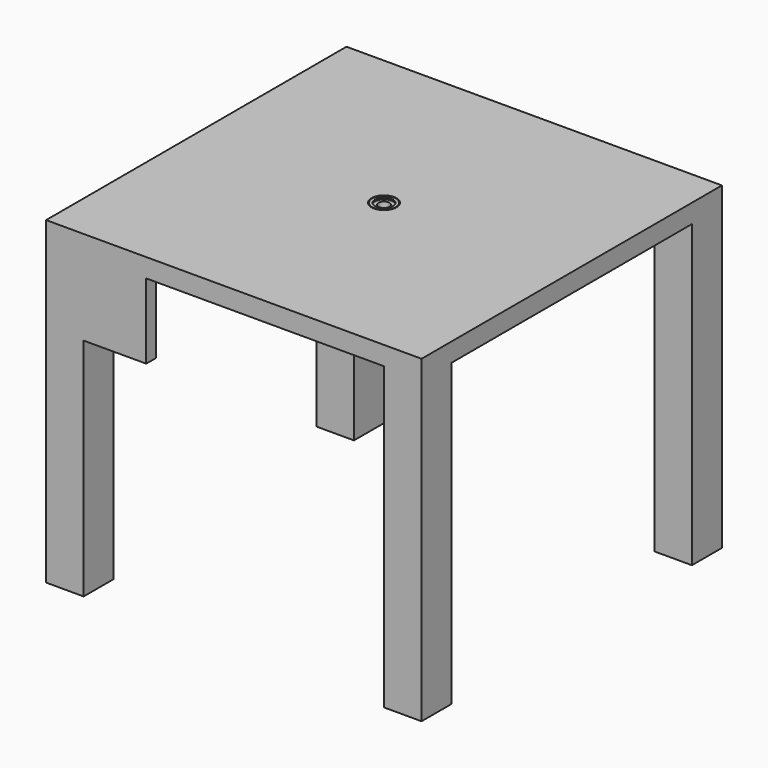
from build123d import *

# Parameters (mm, degrees)
F0_W      = 762
F0_H      = 762
F1_DEPTH  = 38.1
F2_W      = 76.2
F2_H      = 76.2
F3_DEPTH  = 609.6
F4_R      = 18.25625
F5_DEPTH  = 3.60934
F6_R      = 11.1125
F7_DEPTH  = 644.09166
F9_R      = 25.4
F9_R_2    = 23.8125
F10_DEPTH = 12.7
F11_W     = 127
F11_H     = 152.4
F12_DEPTH = 25.4


# Not quite as in the source:
# - a feature of the source that left no trace in its solid (it failed there, or was rolled back) is left out


with BuildPart() as f1:
    # F0 (on Top) → F1 (new body)
    with BuildSketch(Plane.XY):
        Rectangle(F0_W, F0_H)
    extrude(amount=F1_DEPTH)

    # F2 (on face) → F3 (join)
    with BuildSketch(Plane(origin=(0, 0, 0), x_dir=(1, 0, 0), z_dir=(0, 0, -1))):
        with Locations((-342.9, 342.9)):
            Rectangle(F2_W, F2_H)
        with Locations((342.9, 342.9)):
            Rectangle(F2_W, F2_H)
        with Locations((342.9, -342.9)):
            Rectangle(F2_W, F2_H)
        with Locations((-342.9, -342.9)):
            Rectangle(F2_W, F2_H)
    extrude(amount=F3_DEPTH)

    # F4 (on face) → F5 (cut)
    with BuildSketch(Plane.XY.offset(38.1)):
        Circle(F4_R)
    extrude(amount=-F5_DEPTH, mode=Mode.SUBTRACT)

    # F6 (on face) → F7 (cut, through all)
    with BuildSketch(Plane.XY.offset(34.49066)):
        Circle(F6_R)
    extrude(amount=-F7_DEPTH, mode=Mode.SUBTRACT)

    # F9 (on face) → F10 (cut)
    with BuildSketch(Plane.XY.offset(38.1)):
        Circle(F9_R)
        Circle(F9_R_2, mode=Mode.SUBTRACT)
    extrude(amount=-F10_DEPTH, mode=Mode.SUBTRACT)

    # F11 (on face) → F12 (join)
    with BuildSketch(Plane.XZ.offset(381)):
        with Locations((-241.3, -76.2)):
            Rectangle(F11_W, F11_H)
    extrude(amount=-F12_DEPTH)


solid = f1.part
